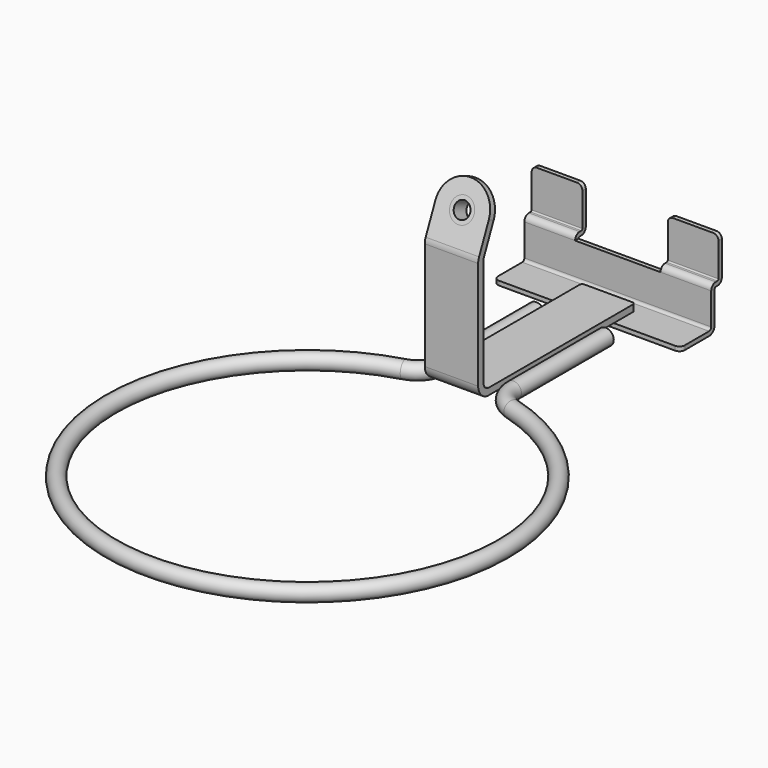
from build123d import *

# Parameters (mm, degrees)
F2_R      = 3
F5_DEPTH  = 10
F6_R      = 9.99999
F7_R      = 4.5
F8_DEPTH  = 87.4178290219
F9_R      = 1
F11_DEPTH = 35
F12_W     = 32
F12_H     = 17.1
F13_DEPTH = 25
F14_R     = 2


# Not quite as in the source:
# - a fillet or chamfer is up to 0.001 mm smaller than in the source, because OpenCascade refuses the exact size


with BuildPart() as f3:
    # F3: sweep along a path in F0
    with BuildLine(Plane.XY) as f3_path:
        Line((13, 123.5), (13, 80.2698573563))
        ThreePointArc((13, 80.2698573563), (15.0142342202, 74.2509251495), (20.245508982, 70.6567007867))
        ThreePointArc((20.245508982, 70.6567007867), (0, -73.5), (-20.245508982, 70.6567007867))
        ThreePointArc((-20.245508982, 70.6567007867), (-15.0142342202, 74.2509251495), (-13, 80.2698573563))
        Line((-13, 80.2698573563), (-13, 123.5))
    # F2 (on plane+point) → F3 (sweep)
    with BuildSketch(Plane.XZ.offset(-123.5)):
        with Locations((13, 0)):
            Circle(F2_R)
    sweep(path=f3_path.line)


with BuildPart() as f5:
    # F4 (on Right) → F5 (new body, symmetric)
    with BuildSketch(Plane.YZ):
        with BuildLine():
            Line((141, 3), (72.5, 3))
            ThreePointArc((72.5, 3), (70.732233047, 3.732233047), (70, 5.5))
            Line((70, 5.5), (70, 45.9747939576))
            ThreePointArc((70, 45.9747939576), (70.0534068222, 46.4887801657), (70.2113454577, 46.9808060778))
            Line((70.2113454577, 46.9808060778), (78.7886545423, 66.4939878798))
            Line((78.7886545423, 66.4939878798), (76.5, 67.5))
            Line((76.5, 67.5), (67.9226909154, 47.9868181981))
            ThreePointArc((67.9226909154, 47.9868181981), (67.6068136443, 47.0027663738), (67.5, 45.9747939576))
            Line((67.5, 45.9747939576), (67.5, 5.5))
            ThreePointArc((67.5, 5.5), (68.9644660941, 1.9644660941), (72.5, 0.5))
            Line((72.5, 0.5), (141, 0.5))
            Line((141, 0.5), (141, 3))
        make_face()
    extrude(amount=F5_DEPTH, both=True)

    # F6 (radius 10 in the source; OpenCascade refuses exactly that, so slightly less here)
    f6_edges = [f5.edges().sort_by_distance(p)[0] for p in [
        (10, 77.644327, 66.996994),
        (-10, 77.644327, 66.996994),
    ]]
    fillet(f6_edges, radius=F6_R)

    # F7 (on face) → F8 (cut, through all)
    with BuildSketch(Plane(origin=(0, 39.2463074221, -17.2512977435), x_dir=(1, 0, 0), z_dir=(0, -0.9154618169, 0.4024048481))):
        with Locations((0, 82.577643521)):
            Circle(F7_R)
    extrude(amount=-F8_DEPTH, mode=Mode.SUBTRACT)

    # F9
    f9_edges = [f5.edges().sort_by_distance(p)[0] for p in [
        (-10, 141, 1.75),
        (10, 141, 1.75),
    ]]
    fillet(f9_edges, radius=F9_R)

    # F10 (on Right) → F11 (join, symmetric)
    with BuildSketch(Plane.YZ):
        with BuildLine():
            Line((144.4, 0.5), (131, 0.5))
            Line((131, 0.5), (131, -1.1))
            Line((131, -1.1), (144.4, -1.1))
            ThreePointArc((144.4, -1.1), (146.2384776311, -0.3384776311), (147, 1.5))
            Line((147, 1.5), (147, 13.4))
            ThreePointArc((147, 13.4), (147.1464466094, 13.7535533906), (147.5, 13.9))
            Line((147.5, 13.9), (148.3, 13.9))
            ThreePointArc((148.3, 13.9), (149.7849242405, 14.5150757595), (150.4, 16))
            Line((150.4, 16), (150.4, 30.5))
            Line((150.4, 30.5), (148.8, 30.5))
            Line((148.8, 30.5), (148.8, 16))
            ThreePointArc((148.8, 16), (148.6535533906, 15.6464466094), (148.3, 15.5))
            Line((148.3, 15.5), (147.5, 15.5))
            ThreePointArc((147.5, 15.5), (146.0150757595, 14.8849242405), (145.4, 13.4))
            Line((145.4, 13.4), (145.4, 1.5))
            ThreePointArc((145.4, 1.5), (145.1071067812, 0.7928932188), (144.4, 0.5))
        make_face()
    extrude(amount=F11_DEPTH, both=True)

    # F12 (on face) → F13 (cut)
    with BuildSketch(Plane.XZ.offset(-145.4)):
        with Locations((0, 21.95)):
            Rectangle(F12_W, F12_H)
    extrude(amount=-F13_DEPTH, mode=Mode.SUBTRACT)

    # F14
    f14_edges = [f5.edges().sort_by_distance(p)[0] for p in [
        (-16, 149.6, 30.5),
        (-35, 149.6, 30.5),
        (16, 149.6, 30.5),
        (35, 149.6, 30.5),
        (-35, 131, -0.3),
        (35, 131, -0.3),
    ]]
    fillet(f14_edges, radius=F14_R)

    # F15 (on Right) → F16 (revolve)
    with BuildSketch(Plane.YZ):
        Polygon((76.5754278778, 61.4589478867), (74.2867733355, 62.464960007), (73.6831660633, 61.0917672816), (79.6336678733, 58.476135769), (80.6396799935, 60.7647903113), (76.9778327259, 62.3744097036), align=None)
    revolve(axis=Axis((0, 74.857979277, 57.2983261259), (0, 0.9154618169, -0.4024048481)))


solid = Compound([f3.part, f5.part])
